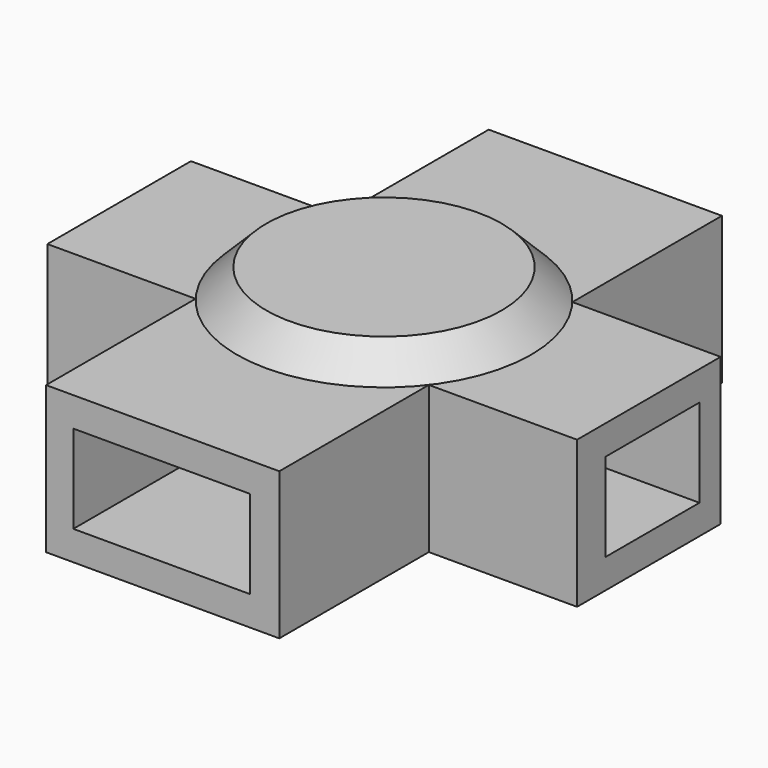
from build123d import *

# Parameters (mm, degrees)
F0_R      = 25
F1_DEPTH  = 30
F0_W      = 90
F0_H      = 94
F2_DEPTH  = 25
F3_SIZE   = 4.99999
F4_W      = 25.1866029114
F4_H      = 31.7543679761
F5_DEPTH  = 100
F6_DEPTH  = 100
F7_W      = 30
F7_H      = 15
F8_DEPTH  = 1000
F9_W      = 20
F9_H      = 15
F10_DEPTH = 100


# Not quite as in the source:
# - a fillet or chamfer is up to 0.001 mm smaller than in the source, because OpenCascade refuses the exact size


with BuildPart() as f1:
    # F0 (on Top) → F1 (new body)
    with BuildSketch(Plane.XY):
        with Locations((16.9619322568, -28.2926298678)):
            Circle(F0_R)
    extrude(amount=F1_DEPTH)

    # F0 (on Top) → F2 (join)
    with BuildSketch(Plane.XY):
        with Locations((16.9619322568, -28.2926298678)):
            Rectangle(F0_W, F0_H)
        with Locations((16.9619322568, -28.2926298678)):
            Circle(F0_R, mode=Mode.SUBTRACT)
    extrude(amount=F2_DEPTH)

    # F3 (size 5 in the source; OpenCascade refuses exactly that, so slightly less here)
    f3_edges = [f1.edges().sort_by_distance(p)[0] for p in [
        (-8.038068, -28.29263, 30),
    ]]
    chamfer(f3_edges, length=F3_SIZE)

    # F4 (on face) → F5 (cut)
    with BuildSketch(Plane.XY.offset(25)):
        with Locations((49.3686308011, 2.8301861442)):
            Rectangle(F4_W, F4_H)
    extrude(amount=-F5_DEPTH, mode=Mode.SUBTRACT)

    # F4 (on face) → F6 (cut)
    with BuildSketch(Plane.XY.offset(25)):
        with Locations((-15.4447662875, 2.8301861442)):
            Rectangle(F4_W, F4_H)
        with Locations((-15.4447662875, -59.4154458798)):
            Rectangle(F4_W, F4_H)
        with Locations((49.3686308011, -59.4154458798)):
            Rectangle(F4_W, F4_H)
    extrude(amount=-F6_DEPTH, mode=Mode.SUBTRACT)

    # F7 (on face) → F8 (cut)
    with BuildSketch(Plane(origin=(0, 18.7073701322, 0), x_dir=(-1, 0, 0), z_dir=(0, 1, 0))):
        with Locations((-16.7753293454, 12.5)):
            Rectangle(F7_W, F7_H)
    extrude(amount=-F8_DEPTH, mode=Mode.SUBTRACT)

    # F9 (on face) → F10 (cut)
    with BuildSketch(Plane.YZ.offset(61.9619322568)):
        with Locations((-27.5469978439, 12.5)):
            Rectangle(F9_W, F9_H)
    extrude(amount=-F10_DEPTH, mode=Mode.SUBTRACT)


solid = f1.part
